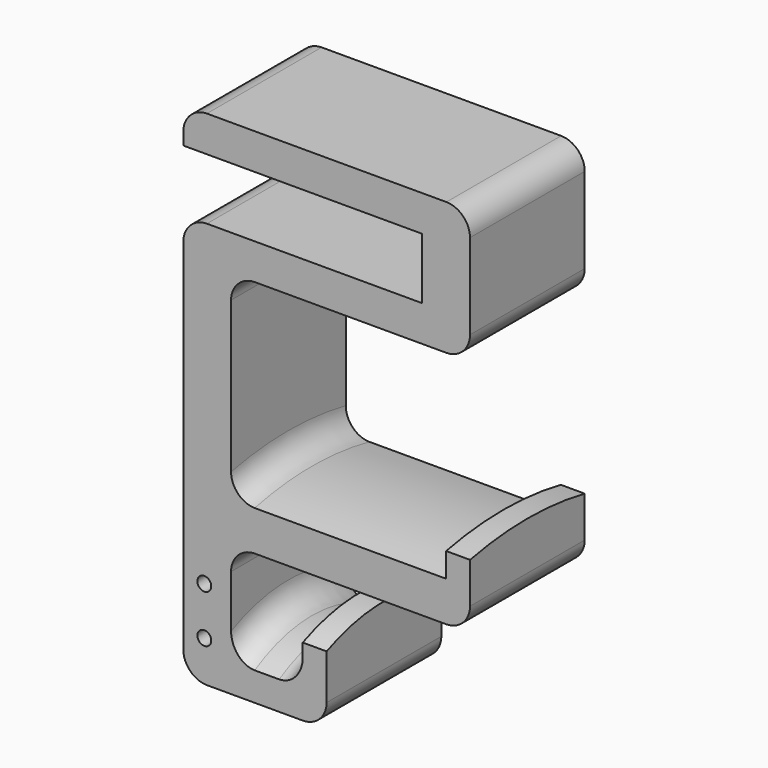
from build123d import *

# Parameters (mm, degrees)
F1_DEPTH     = 19.05
F6_T1_DEPTH  = 38.1
F6_T3_DEPTH  = 19.05
F6_T5_DEPTH  = 19.05
F6_T10_ANGLE = 45.2137620144
F6_T16_ANGLE = 107.7622686142
F6_T22_ANGLE = 107.7622686142
F6_T25_DEPTH = 69.8548284901
F7_R         = 1.8415
F8_DEPTH     = 38.1010001


# Not quite as in the source:
# - a fillet or chamfer that OpenCascade refuses, or shapes differently, is made with other operations: its cross-section is extruded or revolved along the edge and cut away or added


with BuildPart() as f1:
    # F0 (on Front) → F1 (new body, symmetric)
    with BuildSketch(Plane.XZ):
        Polygon((-63.5, 0), (0, 0), (0, -16.2306), (-63.5, -16.2306), (-63.5, -124.1806), (-25.4, -124.1806), (-25.4, -101.9556), (-31.75, -101.9556), (-31.75, -111.4806), (-50.8, -111.4806), (-50.8, -89.2556), (12.7, -89.2556), (12.7, -70.2056), (6.35, -70.2056), (6.35, -76.5556), (-50.8, -76.5556), (-50.8, -25.7556), (12.7, -25.7556), (12.7, 9.525), (-63.5, 9.525), align=None)
    extrude(amount=F1_DEPTH, both=True)

    # F2 (on Front) → F3 (revolve, cut)
    with BuildSketch(Plane.XZ):
        Polygon((-50.8, -57.5056), (-50.8, -76.5556), (6.35, -76.5556), (6.35, -70.2056), (12.7, -70.2056), (12.7, -57.5056), align=None)
    revolve(axis=Axis((-20.4399991781, 0, -165.4556), (1, 0, 0)), mode=Mode.SUBTRACT)

    # F4 (on Front) → F5 (revolve, cut)
    with BuildSketch(Plane.XZ):
        Polygon((-50.8, -89.2556), (-50.8, -111.4806), (-31.75, -111.4806), (-31.75, -101.9556), (-25.4, -101.9556), (-25.4, -89.2556), align=None)
    revolve(axis=Axis((-41.275, 0, -149.5806), (1, 0, 0)), mode=Mode.SUBTRACT)

    # F6: fillet of radius 6.35 on 13 edges, made by hand

    # F6_s2 → F6_t1 (join)
    with BuildSketch(Plane.XZ.offset(-19.05)):
        with BuildLine():
            ThreePointArc((-44.4490343146, -25.7552), (-48.9401280605, -27.6154719395), (-50.8004, -32.1065656854))
            Line((-50.8004, -32.1065656854), (-51.4355365685, -32.1065656854))
            ThreePointArc((-51.4355365685, -32.1065656854), (-51.4351365685, -28.9310828427), (-51.4351365685, -25.7556))
            Line((-51.4351365685, -25.7556), (-50.8, -25.1204634315))
            ThreePointArc((-50.8, -25.1204634315), (-47.6245171573, -25.1204634315), (-44.4490343146, -25.1200634315))
            Line((-44.4490343146, -25.1200634315), (-44.4490343146, -25.7552))
        make_face()
    extrude(amount=F6_T1_DEPTH)

    # F6_s4 → F6_t3 (join)
    with BuildSketch(Plane.XZ.offset(-19.05)):
        with BuildLine():
            ThreePointArc((-44.4490343146, -89.2552), (-48.9401280605, -91.1154719395), (-50.8004, -95.6065656854))
            Line((-50.8004, -95.6065656854), (-51.4355365685, -95.6065656854))
            ThreePointArc((-51.4355365685, -95.6065656854), (-51.4351365685, -92.4310828427), (-51.4351365685, -89.2556))
            Line((-51.4351365685, -89.2556), (-50.8, -88.6204634315))
            ThreePointArc((-50.8, -88.6204634315), (-47.6245171573, -88.6204634315), (-44.4490343146, -88.6200634315))
            Line((-44.4490343146, -88.6200634315), (-44.4490343146, -89.2552))
        make_face()
    extrude(amount=F6_T3_DEPTH)

    # F6_s6 → F6_t5 (join)
    with BuildSketch(Plane.XZ):
        with BuildLine():
            ThreePointArc((-44.4490343146, -89.2552), (-48.9401280605, -91.1154719395), (-50.8004, -95.6065656854))
            Line((-50.8004, -95.6065656854), (-51.4355365685, -95.6065656854))
            ThreePointArc((-51.4355365685, -95.6065656854), (-51.4351365685, -92.4310828427), (-51.4351365685, -89.2556))
            Line((-51.4351365685, -89.2556), (-50.8, -88.6204634315))
            ThreePointArc((-50.8, -88.6204634315), (-47.6245171573, -88.6204634315), (-44.4490343146, -88.6200634315))
            Line((-44.4490343146, -88.6200634315), (-44.4490343146, -89.2552))
        make_face()
    extrude(amount=F6_T5_DEPTH)


with BuildPart() as f6_tool8:
    # F6_s9 → F6_t10 (revolve)
    with BuildSketch(Plane(origin=(0, -58.7152257849, -24.4490632784), x_dir=(1, 0, 0), z_dir=(0, -0.923164058, -0.384406194))):
        with BuildLine():
            ThreePointArc((-50.8004, -57.4916974353), (-48.9401280605, -61.9827911812), (-44.4490343146, -63.8430631207))
            Line((-44.4490343146, -63.8430631207), (-44.4490343146, -64.4781996892))
            ThreePointArc((-44.4490343146, -64.4781996892), (-47.6245171573, -64.4777996892), (-50.8, -64.4777996892))
            Line((-50.8, -64.4777996892), (-51.4351365685, -63.8426631207))
            ThreePointArc((-51.4351365685, -63.8426631207), (-51.4351365685, -60.667180278), (-51.4355365685, -57.4916974353))
            Line((-51.4355365685, -57.4916974353), (-50.8004, -57.4916974353))
        make_face()
    revolve(axis=Axis((-50.8, 0, -165.4556), (-1, 0, 0)), revolution_arc=F6_T10_ANGLE)

    split(bisect_by=Plane.XZ.offset(19.05), keep=Keep.BOTTOM)

    split(bisect_by=Plane.XZ.offset(-19.05), keep=Keep.TOP)


with BuildPart() as f1_1:
    add(f1.part)

    # F6_t7: union F6_tool8
    add(f6_tool8.part)


with BuildPart() as f6_tool14:
    # F6_s15 → F6_t16 (revolve)
    with BuildSketch(Plane(origin=(0, -71.2250836382, -97.6064441708), x_dir=(1, 0, 0), z_dir=(0, -0.589462371, -0.8077958363))):
        with BuildLine():
            ThreePointArc((-50.8004, -43.7211694448), (-48.9401280605, -48.2122631908), (-44.4490343146, -50.0725351302))
            Line((-44.4490343146, -50.0725351302), (-44.4490343146, -50.7076716988))
            ThreePointArc((-44.4490343146, -50.7076716988), (-47.6245171573, -50.7072716988), (-50.8, -50.7072716988))
            Line((-50.8, -50.7072716988), (-51.4351365685, -50.0721351302))
            ThreePointArc((-51.4351365685, -50.0721351302), (-51.4351365685, -46.8966522875), (-51.4355365685, -43.7211694448))
            Line((-51.4355365685, -43.7211694448), (-50.8004, -43.7211694448))
        make_face()
    revolve(axis=Axis((-50.8, 0, -149.5806), (-1, 0, 0)), revolution_arc=F6_T16_ANGLE)

    split(bisect_by=Plane.XZ.offset(19.05), keep=Keep.BOTTOM)

    split(bisect_by=Plane.XZ.offset(-19.05), keep=Keep.TOP)


with BuildPart() as f1_2:
    add(f1_1.part)

    # F6_t13: union F6_tool14
    add(f6_tool14.part)


with BuildPart() as f6_tool20:
    # F6_s21 → F6_t22 (revolve)
    with BuildSketch(Plane(origin=(0, -71.2250836382, -97.6064441708), x_dir=(1, 0, 0), z_dir=(0, -0.589462371, -0.8077958363))):
        with BuildLine():
            ThreePointArc((-38.1009656854, -50.0725351302), (-33.6098719395, -48.2122631908), (-31.7496, -43.7211694448))
            Line((-31.7496, -43.7211694448), (-31.1144634315, -43.7211694448))
            ThreePointArc((-31.1144634315, -43.7211694448), (-31.1148634315, -46.8966522875), (-31.1148634315, -50.0721351302))
            Line((-31.1148634315, -50.0721351302), (-31.75, -50.7072716988))
            ThreePointArc((-31.75, -50.7072716988), (-34.9254828427, -50.7072716988), (-38.1009656854, -50.7076716988))
            Line((-38.1009656854, -50.7076716988), (-38.1009656854, -50.0725351302))
        make_face()
    revolve(axis=Axis((-31.75, 0, -149.5806), (-1, 0, 0)), revolution_arc=F6_T22_ANGLE)

    split(bisect_by=Plane.XZ.offset(19.05), keep=Keep.BOTTOM)

    split(bisect_by=Plane.XZ.offset(-19.05), keep=Keep.TOP)


with BuildPart() as f1_3:
    add(f1_2.part)

    # F6_t19: union F6_tool20
    add(f6_tool20.part)

    # F6_s26 → F6_t25 (cut)
    with BuildSketch(Plane.XZ.offset(-34.9274142451)):
        with BuildLine():
            ThreePointArc((6.3490343146, 9.5254), (10.8401280605, 7.6651280605), (12.7004, 3.1740343146))
            Line((12.7004, 3.1740343146), (13.3355365685, 3.1740343146))
            ThreePointArc((13.3355365685, 3.1740343146), (13.3351365685, 6.3495171573), (13.3351365685, 9.525))
            Line((13.3351365685, 9.525), (12.7, 10.1601365685))
            ThreePointArc((12.7, 10.1601365685), (9.5245171573, 10.1601365685), (6.3490343146, 10.1605365685))
            Line((6.3490343146, 10.1605365685), (6.3490343146, 9.5254))
        make_face()
        with BuildLine():
            ThreePointArc((-57.1490343146, 9.5254), (-61.6401280605, 7.6651280605), (-63.5004, 3.1740343146))
            Line((-63.5004, 3.1740343146), (-64.1355365685, 3.1740343146))
            ThreePointArc((-64.1355365685, 3.1740343146), (-64.1351365685, 6.3495171573), (-64.1351365685, 9.525))
            Line((-64.1351365685, 9.525), (-63.5, 10.1601365685))
            ThreePointArc((-63.5, 10.1601365685), (-60.3245171573, 10.1601365685), (-57.1490343146, 10.1605365685))
            Line((-57.1490343146, 10.1605365685), (-57.1490343146, 9.5254))
        make_face()
        with BuildLine():
            ThreePointArc((-63.5004, -22.5815656854), (-61.6401280605, -18.0904719395), (-57.1490343146, -16.2302))
            Line((-57.1490343146, -16.2302), (-57.1490343146, -15.5950634315))
            ThreePointArc((-57.1490343146, -15.5950634315), (-60.3245171573, -15.5954634315), (-63.5, -15.5954634315))
            Line((-63.5, -15.5954634315), (-64.1351365685, -16.2306))
            ThreePointArc((-64.1351365685, -16.2306), (-64.1351365685, -19.4060828427), (-64.1355365685, -22.5815656854))
            Line((-64.1355365685, -22.5815656854), (-63.5004, -22.5815656854))
        make_face()
        with BuildLine():
            ThreePointArc((12.7004, -19.4046343146), (10.8401280605, -23.8957280605), (6.3490343146, -25.756))
            Line((6.3490343146, -25.756), (6.3490343146, -26.3911365685))
            ThreePointArc((6.3490343146, -26.3911365685), (9.5245171573, -26.3907365685), (12.7, -26.3907365685))
            Line((12.7, -26.3907365685), (13.3351365685, -25.7556))
            ThreePointArc((13.3351365685, -25.7556), (13.3351365685, -22.5801171573), (13.3355365685, -19.4046343146))
            Line((13.3355365685, -19.4046343146), (12.7004, -19.4046343146))
        make_face()
        with BuildLine():
            ThreePointArc((-57.1490343146, -124.181), (-61.6401280605, -122.3207280605), (-63.5004, -117.8296343146))
            Line((-63.5004, -117.8296343146), (-64.1355365685, -117.8296343146))
            ThreePointArc((-64.1355365685, -117.8296343146), (-64.1351365685, -121.0051171573), (-64.1351365685, -124.1806))
            Line((-64.1351365685, -124.1806), (-63.5, -124.8157365685))
            ThreePointArc((-63.5, -124.8157365685), (-60.3245171573, -124.8157365685), (-57.1490343146, -124.8161365685))
            Line((-57.1490343146, -124.8161365685), (-57.1490343146, -124.181))
        make_face()
        with BuildLine():
            ThreePointArc((-25.3996, -117.8296343146), (-27.2598719395, -122.3207280605), (-31.7509656854, -124.181))
            Line((-31.7509656854, -124.181), (-31.7509656854, -124.8161365685))
            ThreePointArc((-31.7509656854, -124.8161365685), (-28.5754828427, -124.8157365685), (-25.4, -124.8157365685))
            Line((-25.4, -124.8157365685), (-24.7648634315, -124.1806))
            ThreePointArc((-24.7648634315, -124.1806), (-24.7648634315, -121.0051171573), (-24.7644634315, -117.8296343146))
            Line((-24.7644634315, -117.8296343146), (-25.3996, -117.8296343146))
        make_face()
        with BuildLine():
            ThreePointArc((12.7004, -82.9046343146), (10.8401280605, -87.3957280605), (6.3490343146, -89.256))
            Line((6.3490343146, -89.256), (6.3490343146, -89.8911365685))
            ThreePointArc((6.3490343146, -89.8911365685), (9.5245171573, -89.8907365685), (12.7, -89.8907365685))
            Line((12.7, -89.8907365685), (13.3351365685, -89.2556))
            ThreePointArc((13.3351365685, -89.2556), (13.3351365685, -86.0801171573), (13.3355365685, -82.9046343146))
            Line((13.3355365685, -82.9046343146), (12.7004, -82.9046343146))
        make_face()
    extrude(amount=F6_T25_DEPTH, mode=Mode.SUBTRACT)

    # F7 (on face) → F8 (cut, through all)
    with BuildSketch(Plane.XZ.offset(19.05)):
        with Locations((-57.9040207225, -100.6856)):
            Circle(F7_R)
        with Locations((-57.9040207225, -113.3856)):
            Circle(F7_R)
    extrude(amount=-F8_DEPTH, mode=Mode.SUBTRACT)


solid = f1_3.part
